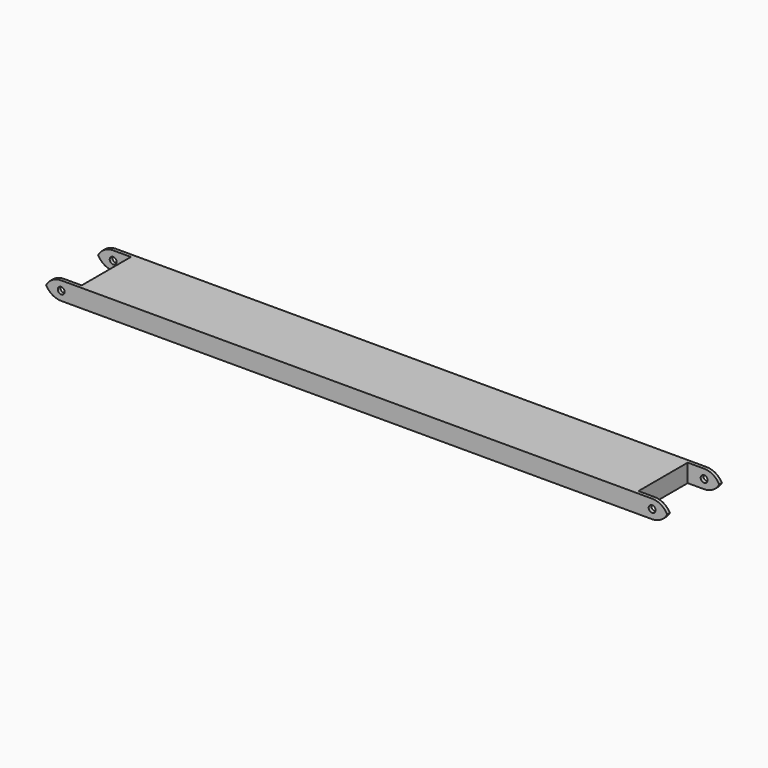
from build123d import *

# Parameters (mm, degrees)
F0_W        = 182.7820166945
F0_H        = 5.2849859931
F1_DEPTH    = 20
F2_T1_DEPTH = 45
F3_D        = 2
F4_T1_DEPTH = 45
F5_D        = 2
F6_W        = 10.6622725725
F6_H        = 5.6903085506
F9_DEPTH    = 18
F6_W_2      = 10.1688206196
F6_H_2      = 8.087759139
F10_DEPTH   = 18


# Not quite as in the source:
# - a fillet or chamfer that OpenCascade refuses, or shapes differently, is made with other operations: its cross-section is extruded or revolved along the edge and cut away or added


with BuildPart() as f1:
    # F0 (on Front) → F1 (new body)
    with BuildSketch(Plane.XZ):
        with Locations((16.4561159909, 2.6424929965)):
            Rectangle(F0_W, F0_H)
    extrude(amount=-F1_DEPTH)

    # F2: fillet of radius 5 on 2 edges, made by hand

    # F2_s2 → F2_t1 (cut)
    with BuildSketch(Plane.XZ.offset(-32.5)):
        with BuildLine():
            ThreePointArc((-74.9348923564, 0.2849859931), (-73.4704262623, 3.820519899), (-69.9348923564, 5.2849859931))
            Line((-69.9348923564, 5.2849859931), (-74.9348923564, 5.2849859931))
            Line((-74.9348923564, 5.2849859931), (-74.9348923564, 0.2849859931))
        make_face()
        with BuildLine():
            ThreePointArc((-74.9348923564, 5), (-73.4704262623, 1.4644660941), (-69.9348923564, 0))
            Line((-69.9348923564, 0), (-74.9348923564, 0))
            Line((-74.9348923564, 0), (-74.9348923564, 5))
        make_face()
    extrude(amount=F2_T1_DEPTH, mode=Mode.SUBTRACT)

    # F3 (through all)
    with Locations(Plane.XZ):
        with Locations((-69.9340328574, 2.630488947)):
            Hole(F3_D / 2)

    # F4: fillet of radius 5 on 2 edges, made by hand

    # F4_s2 → F4_t1 (cut)
    with BuildSketch(Plane.XZ.offset(-32.5)):
        with BuildLine():
            ThreePointArc((102.8471243382, 5.2849859931), (106.3826582441, 3.820519899), (107.8471243382, 0.2849859931))
            Line((107.8471243382, 0.2849859931), (107.8471243382, 5.2849859931))
            Line((107.8471243382, 5.2849859931), (102.8471243382, 5.2849859931))
        make_face()
        with BuildLine():
            ThreePointArc((107.8471243382, 5), (106.3826582441, 1.4644660941), (102.8471243382, 0))
            Line((102.8471243382, 0), (107.8471243382, 0))
            Line((107.8471243382, 0), (107.8471243382, 5))
        make_face()
    extrude(amount=F4_T1_DEPTH, mode=Mode.SUBTRACT)

    # F5 (through all)
    with Locations(Plane.XZ):
        with Locations((102.8473824263, 2.641917672)):
            Hole(F5_D / 2)


with BuildPart() as f1_1:
    # F7: moved
    add(f1.part.moved(Location((-1, 1, 0))))


with BuildPart() as f1_2:
    # F8: moved
    add(f1_1.part.moved(Location((0, -2, 0))))

    # F6 (on Front) → F9 (cut)
    with BuildSketch(Plane.XZ):
        with Locations((-71.0640922189, 2.8451542753)):
            Rectangle(F6_W, F6_H)
    extrude(amount=-F9_DEPTH, mode=Mode.SUBTRACT)

    # F6 (on Front) → F10 (cut)
    with BuildSketch(Plane.XZ):
        with Locations((102.1384820342, 2.511022496)):
            Rectangle(F6_W_2, F6_H_2)
    extrude(amount=-F10_DEPTH, mode=Mode.SUBTRACT)


solid = f1_2.part
